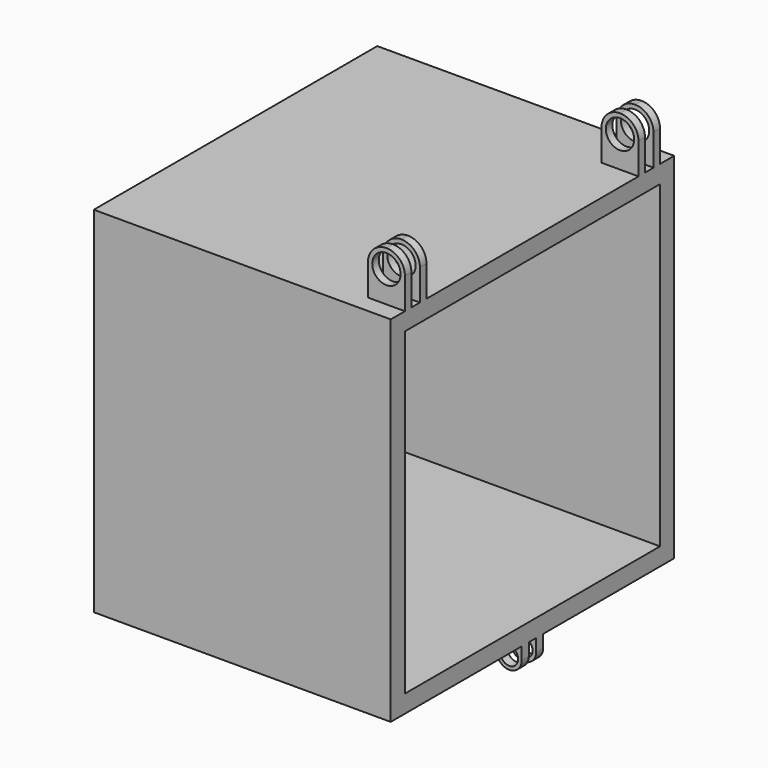
from build123d import *

# Parameters (mm, degrees)
F0_W      = 127
F0_H      = 127
F0_W_2    = 114.3
F0_H_2    = 114.3
F1_DEPTH  = 106.426
F2_W      = 127
F2_H      = 127
F3_DEPTH  = 6.35
F4_W      = 13.2588
F4_H      = 9.652
F5_DEPTH  = 17.78
F6_W      = 3.81
F6_H      = 17.78
F7_DEPTH  = 106.427
F8_R      = 6.62939
F9_R      = 5.08
F10_DEPTH = 25.4
F11_W     = 8.89
F11_H     = 3.175
F12_DEPTH = 8.89
F13_R     = 4.44499
F14_R     = 3.175
F15_DEPTH = 25.4


# Not quite as in the source:
# - a fillet or chamfer is up to 0.001 mm smaller than in the source, because OpenCascade refuses the exact size
# - a pattern or mirror of a feature is missing from the dataset's text; its kind, count and spacing are read off the source's solid


with BuildPart() as f1:
    # F0 (on Right) → F1 (new body)
    with BuildSketch(Plane.YZ):
        Rectangle(F0_W, F0_H)
        Rectangle(F0_W_2, F0_H_2, mode=Mode.SUBTRACT)
    extrude(amount=F1_DEPTH)

    # F2 (on Right) → F3 (join)
    with BuildSketch(Plane.YZ):
        Rectangle(F2_W, F2_H)
    extrude(amount=F3_DEPTH)

    # F4 (on face) → F5 (join)
    with BuildSketch(Plane.XY.offset(63.5)):
        with Locations((99.7966, 52.324)):
            Rectangle(F4_W, F4_H)
    f5 = extrude(amount=F5_DEPTH)

    # F5_copies: F5 across plane
    add(f5.mirror(Plane(origin=(0, 3e-06, 0), x_dir=(0, 0, -1), z_dir=(0, -1, 0))))

    # F6 (on face) → F7 (cut, through all)
    with BuildSketch(Plane.YZ.offset(106.426)):
        with Locations((52.324, 72.39)):
            Rectangle(F6_W, F6_H)
    f7 = extrude(amount=-F7_DEPTH, mode=Mode.SUBTRACT)

    # F7_copies: F7 across plane
    add(f7.mirror(Plane(origin=(0, 2e-06, 0), x_dir=(0, 0, -1), z_dir=(0, -1, 0))), mode=Mode.SUBTRACT)

    # F8 (radius 6.6294 in the source; OpenCascade refuses exactly that, so slightly less here)
    f8_edges = [f1.edges().sort_by_distance(p)[0] for p in [
        (106.426, 55.6895, 81.28),
        (106.426, 48.9585, 81.28),
        (93.1672, 55.6895, 81.28),
        (93.1672, 48.9585, 81.28),
        (93.1672, -55.689495, 81.28),
        (106.426, -55.689495, 81.28),
        (93.1672, -48.958495, 81.28),
        (106.426, -48.958495, 81.28),
    ]]
    fillet(f8_edges, radius=F8_R)

    # F9 (on face) → F10 (cut)
    with BuildSketch(Plane(origin=(0, 57.15, 0), x_dir=(-1, 0, 0), z_dir=(0, 1, 0))):
        with Locations((-99.7966, 74.6506)):
            Circle(F9_R)
    f10 = extrude(amount=-F10_DEPTH, mode=Mode.SUBTRACT)

    # F10_copies: F10 across plane
    add(f10.mirror(Plane(origin=(0, 0, 0), x_dir=(0, 0, -1), z_dir=(0, -1, 0))), mode=Mode.SUBTRACT)

    # F11 (on face) → F12 (join)
    with BuildSketch(Plane(origin=(0, 0, -63.5), x_dir=(1, 0, 0), z_dir=(0, 0, -1))):
        with Locations((101.981, 3.2385)):
            Rectangle(F11_W, F11_H)
        with Locations((101.981, -3.2385)):
            Rectangle(F11_W, F11_H)
    extrude(amount=F12_DEPTH)

    # F13 (radius 4.445 in the source; OpenCascade refuses exactly that, so slightly less here)
    f13_edges = [f1.edges().sort_by_distance(p)[0] for p in [
        (97.536, -3.2385, -72.39),
        (97.536, 3.2385, -72.39),
        (106.426, 3.2385, -72.39),
        (106.426, -3.2385, -72.39),
    ]]
    fillet(f13_edges, radius=F13_R)

    # F14 (on face) → F15 (cut)
    with BuildSketch(Plane.XZ.offset(4.826)):
        with Locations((101.981, -67.945)):
            Circle(F14_R)
    extrude(amount=-F15_DEPTH, mode=Mode.SUBTRACT)


solid = f1.part
